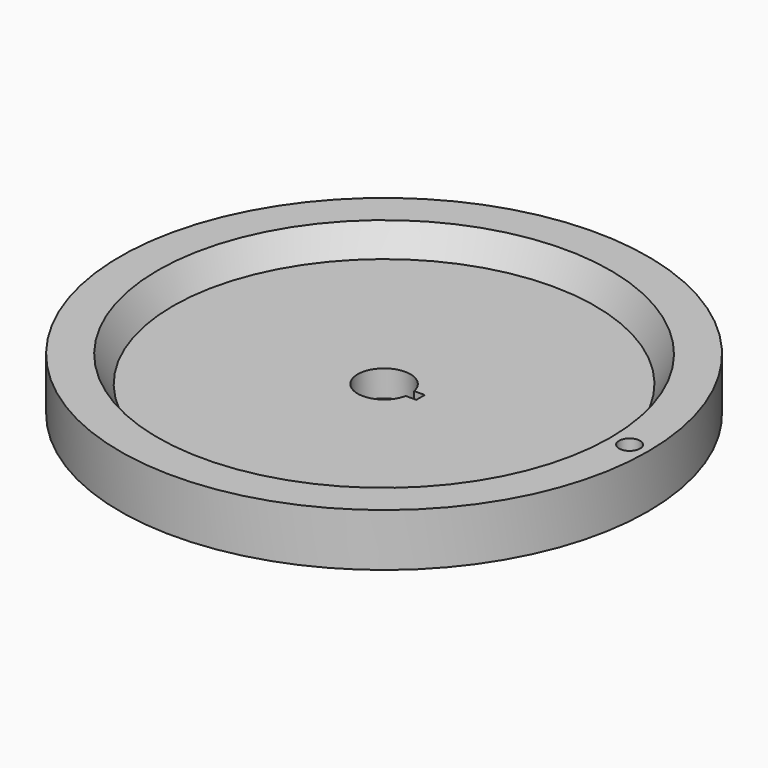
from build123d import *

# Parameters (mm, degrees)
F0_R     = 5
F0_R_2   = 4
F0_R_3   = 0.2
F1_DEPTH = 1
F2_DEPTH = 0.5
F4_DEPTH = 25
F5_SIZE2 = 0.288665
F5_SIZE  = 0.49999


# Not quite as in the source:
# - a fillet or chamfer is up to 0.001 mm smaller than in the source, because OpenCascade refuses the exact size


with BuildPart() as f1:
    # F0 (on Top) → F1 (new body)
    with BuildSketch(Plane.XY):
        Circle(F0_R)
        Circle(F0_R_2, mode=Mode.SUBTRACT)
        with Locations((4.65, 0)):
            Circle(F0_R_3, mode=Mode.SUBTRACT)
    extrude(amount=F1_DEPTH)

    # F0 (on Top) → F2 (join)
    with BuildSketch(Plane.XY):
        Circle(F0_R_2)
    extrude(amount=F2_DEPTH)

    # F3 (on face) → F4 (cut)
    with BuildSketch(Plane.XY.offset(0.5)):
        with BuildLine():
            ThreePointArc((0.4898979486, -0.1), (0.4974680765, -0.050254481), (0.5, 0))
            ThreePointArc((0.5, 0), (0.4974680765, 0.050254481), (0.4898979486, 0.1))
            ThreePointArc((0.4898979486, 0.1), (-0.5, 0), (0.4898979486, -0.1))
        make_face()
        with BuildLine():
            ThreePointArc((0.4898979486, 0.1), (0.4974680765, 0.050254481), (0.5, 0))
            ThreePointArc((0.5, 0), (0.4974680765, -0.050254481), (0.4898979486, -0.1))
            Line((0.4898979486, -0.1), (0.6898979486, -0.1))
            Line((0.6898979486, -0.1), (0.6898979486, 0))
            Line((0.6898979486, 0), (0.6898979486, 0.1))
            Line((0.6898979486, 0.1), (0.4898979486, 0.1))
        make_face()
    extrude(amount=-F4_DEPTH, mode=Mode.SUBTRACT)

    # F5 (size 0.5 and 0.2886751346 in the source; OpenCascade refuses exactly that, so slightly less here)
    f5_edges = [f1.edges().sort_by_distance(p)[0] for p in [
        (-4, 0, 1),
    ]]
    f5_side = f1.faces().sort_by_distance((-4, 0, 0.75))[0]
    chamfer(f5_edges, length=F5_SIZE, length2=F5_SIZE2, reference=f5_side)


solid = f1.part
